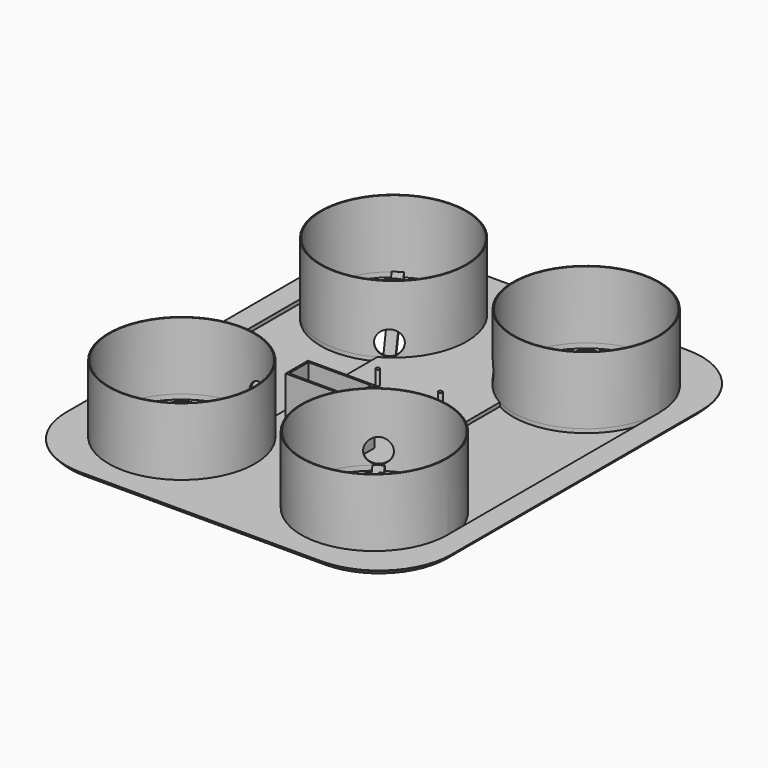
from build123d import *

# Parameters (mm, degrees)
F0_W           = 160
F0_H           = 190
F1_DEPTH       = 2
F2_R           = 30
F4_DEPTH       = 12
F5_R           = 30.4
F5_R_2         = 30
F6_DEPTH       = 30
F9_R           = 5
F10_DEPTH      = 60
F10_DEPTH_BACK = 60
F12_R          = 5
F13_DEPTH      = 50
F13_DEPTH_BACK = 50
F14_R          = 0.8
F15_DEPTH      = 8
F16_W          = 27.6
F16_H          = 11.6
F16_W_2        = 26
F16_H_2        = 10
F17_DEPTH      = 25
F18_SIZE       = 1.8
F20_DEPTH      = 1.6


with BuildPart() as f1:
    # F0 (on Top) → F1 (new body)
    with BuildSketch(Plane.XY):
        Rectangle(F0_W, F0_H)
        with BuildLine():
            Line((-44.944674, -58.398559), (-59.223368, -78.031763))
            ThreePointArc((-59.223368, -78.031763), (-64.262083, -37.354849), (-24.011576, -29.61555))
            Line((-24.011576, -29.61555), (-38.556221, -49.176298))
            ThreePointArc((-38.556221, -49.176298), (-44.932199, -51.583362), (-44.944674, -58.398559))
        make_face(mode=Mode.SUBTRACT)
        with BuildLine():
            ThreePointArc((-20.776632, -31.968237), (-15.737917, -72.645151), (-55.988424, -80.38445))
            Line((-55.988424, -80.38445), (-41.709729, -60.751246))
            ThreePointArc((-41.709729, -60.751246), (-35.229927, -58.639561), (-34.904454, -51.832129))
            Line((-34.904454, -51.832129), (-20.776632, -31.968237))
        make_face(mode=Mode.SUBTRACT)
        with BuildLine():
            ThreePointArc((55.988424, -80.38445), (15.737917, -72.645151), (20.776632, -31.968237))
            Line((20.776632, -31.968237), (35.055326, -51.601441))
            ThreePointArc((35.055326, -51.601441), (35.147583, -58.52903), (41.709729, -60.751246))
            Line((41.709729, -60.751246), (55.988424, -80.38445))
        make_face(mode=Mode.SUBTRACT)
        with BuildLine():
            ThreePointArc((24.011576, -29.61555), (64.262083, -37.354849), (59.223368, -78.031763))
            Line((59.223368, -78.031763), (44.944674, -58.398559))
            ThreePointArc((44.944674, -58.398559), (44.852417, -51.47097), (38.290271, -49.248754))
            Line((38.290271, -49.248754), (24.011576, -29.61555))
        make_face(mode=Mode.SUBTRACT)
        with BuildLine():
            ThreePointArc((-24.011576, 29.61555), (-64.262083, 37.354849), (-59.223368, 78.031763))
            Line((-59.223368, 78.031763), (-44.944674, 58.398559))
            ThreePointArc((-44.944674, 58.398559), (-44.852417, 51.47097), (-38.290271, 49.248754))
            Line((-38.290271, 49.248754), (-24.011576, 29.61555))
        make_face(mode=Mode.SUBTRACT)
        with BuildLine():
            ThreePointArc((-55.988424, 80.38445), (-15.737917, 72.645151), (-20.776632, 31.968237))
            Line((-20.776632, 31.968237), (-35.055326, 51.601441))
            ThreePointArc((-35.055326, 51.601441), (-35.147583, 58.52903), (-41.709729, 60.751246))
            Line((-41.709729, 60.751246), (-55.988424, 80.38445))
        make_face(mode=Mode.SUBTRACT)
        with BuildLine():
            ThreePointArc((20.776632, 31.968237), (15.737917, 72.645151), (55.988424, 80.38445))
            Line((55.988424, 80.38445), (41.709729, 60.751246))
            ThreePointArc((41.709729, 60.751246), (35.147583, 58.52903), (35.055326, 51.601441))
            Line((35.055326, 51.601441), (20.776632, 31.968237))
        make_face(mode=Mode.SUBTRACT)
        with BuildLine():
            Line((44.944674, 58.398559), (59.223368, 78.031763))
            ThreePointArc((59.223368, 78.031763), (64.262083, 37.354849), (24.011576, 29.61555))
            Line((24.011576, 29.61555), (38.290271, 49.248754))
            ThreePointArc((38.290271, 49.248754), (44.852417, 51.47097), (44.944674, 58.398559))
        make_face(mode=Mode.SUBTRACT)
    extrude(amount=F1_DEPTH)

    # F2
    f2_edges = [f1.edges().sort_by_distance(p)[0] for p in [
        (-80, 95, 1),
        (80, 95, 1),
        (80, -95, 1),
        (-80, -95, 1),
    ]]
    fillet(f2_edges, radius=F2_R)

    # F3 (on Top) → F4 (join)
    with BuildSketch(Plane.XY):
        with BuildLine():
            Line((-36.723614, 52.535189), (-35.571787, 50.951428))
            ThreePointArc((-35.571787, 50.951428), (-43.52903, 59.852417), (-37.512754, 49.539816))
            Line((-37.512754, 49.539816), (-38.66458, 51.123577))
            ThreePointArc((-38.66458, 51.123577), (-42.411504, 58.315818), (-36.723614, 52.535189))
        make_face()
        with BuildLine():
            Line((35.571787, 50.951428), (36.723614, 52.535189))
            ThreePointArc((36.723614, 52.535189), (42.411504, 58.315818), (38.66458, 51.123577))
            Line((38.66458, 51.123577), (37.512754, 49.539816))
            ThreePointArc((37.512754, 49.539816), (43.52903, 59.852417), (35.571787, 50.951428))
        make_face()
        with BuildLine():
            Line((36.723614, -52.535189), (35.571787, -50.951428))
            ThreePointArc((35.571787, -50.951428), (43.52903, -59.852417), (37.512754, -49.539816))
            Line((37.512754, -49.539816), (38.66458, -51.123577))
            ThreePointArc((38.66458, -51.123577), (42.411504, -58.315818), (36.723614, -52.535189))
        make_face()
        with BuildLine():
            Line((-35.571787, -50.951428), (-36.723614, -52.535189))
            ThreePointArc((-36.723614, -52.535189), (-42.411504, -58.315818), (-38.66458, -51.123577))
            Line((-38.66458, -51.123577), (-37.512754, -49.539816))
            ThreePointArc((-37.512754, -49.539816), (-43.52903, -59.852417), (-35.571787, -50.951428))
        make_face()
    extrude(amount=F4_DEPTH)

    # F5 (on Top) → F6 (join)
    with BuildSketch(Plane.XY):
        with Locations((-40, 55)):
            Circle(F5_R)
        with Locations((-40, 55)):
            Circle(F5_R_2, mode=Mode.SUBTRACT)
        with Locations((40, 55)):
            Circle(F5_R)
        with Locations((40, 55)):
            Circle(F5_R_2, mode=Mode.SUBTRACT)
        with Locations((-40, -55)):
            Circle(F5_R)
        with Locations((-40, -55)):
            Circle(F5_R_2, mode=Mode.SUBTRACT)
        with Locations((40, -55)):
            Circle(F5_R)
        with Locations((40, -55)):
            Circle(F5_R_2, mode=Mode.SUBTRACT)
    extrude(amount=F6_DEPTH)

    # F9 (on line) → F10 (cut, two sides)
    with BuildSketch(Plane(origin=(0, 0, 0), x_dir=(-0.809017, -0.587785, 0), z_dir=(-0.587785, 0.809017, 0))) as f10_sk:
        with Locations((0, 7.346634)):
            Circle(F9_R)
    extrude(amount=-F10_DEPTH, mode=Mode.SUBTRACT)
    extrude(f10_sk.sketch, amount=F10_DEPTH_BACK, mode=Mode.SUBTRACT)

    # F12 (on line) → F13 (cut, two sides)
    with BuildSketch(Plane(origin=(0, 0, 0), x_dir=(-0.809017, 0.587785, 0), z_dir=(0.587785, 0.809017, 0))) as f13_sk:
        with Locations((8.821786, 8.548897)):
            Circle(F12_R)
    extrude(amount=-F13_DEPTH, mode=Mode.SUBTRACT)
    extrude(f13_sk.sketch, amount=F13_DEPTH_BACK, mode=Mode.SUBTRACT)

    # F14 (on Top) → F15 (join)
    with BuildSketch(Plane.XY):
        with Locations((-13, 13)):
            Circle(F14_R)
        with Locations((13, 13)):
            Circle(F14_R)
        with Locations((-13, -13)):
            Circle(F14_R)
    extrude(amount=F15_DEPTH)

    # F16 (on Top) → F17 (join)
    with BuildSketch(Plane.XY):
        with Locations((0, -28)):
            Rectangle(F16_W, F16_H)
        with Locations((0, -28)):
            Rectangle(F16_W_2, F16_H_2, mode=Mode.SUBTRACT)
    extrude(amount=F17_DEPTH)

    # F18
    f18_edges = [f1.edges().sort_by_distance(p)[0] for p in [
        (80, 0, 0),
        (71.213203, -86.213203, 0),
        (0, -95, 0),
        (-71.213203, -86.213203, 0),
        (-80, 0, 0),
        (-71.213203, 86.213203, 0),
        (0, 95, 0),
        (71.213203, 86.213203, 0),
    ]]
    chamfer(f18_edges, length=F18_SIZE)

    # F19 (on face) → F20 (cut)
    with BuildSketch(Plane.XY.offset(2)):
        with BuildLine():
            ThreePointArc((-25.435597, 28.315957), (-55.455544, 28.822029), (-70.399691, 54.862879))
            Line((-70.399691, 54.862879), (-70.4, -54.999914))
            ThreePointArc((-70.4, -54.999914), (-55.514507, -28.856931), (-25.435597, -28.315957))
            Line((-25.435597, -28.315957), (-25.435597, 28.315957))
        make_face()
        with BuildLine():
            Line((25.435597, 28.315957), (25.435597, -28.315957))
            ThreePointArc((25.435597, -28.315957), (55.514507, -28.856931), (70.4, -54.999914))
            Line((70.4, -54.999914), (70.399691, 54.862879))
            ThreePointArc((70.399691, 54.862879), (55.455544, 28.822029), (25.435597, 28.315957))
        make_face()
    extrude(amount=-F20_DEPTH, mode=Mode.SUBTRACT)


solid = f1.part
